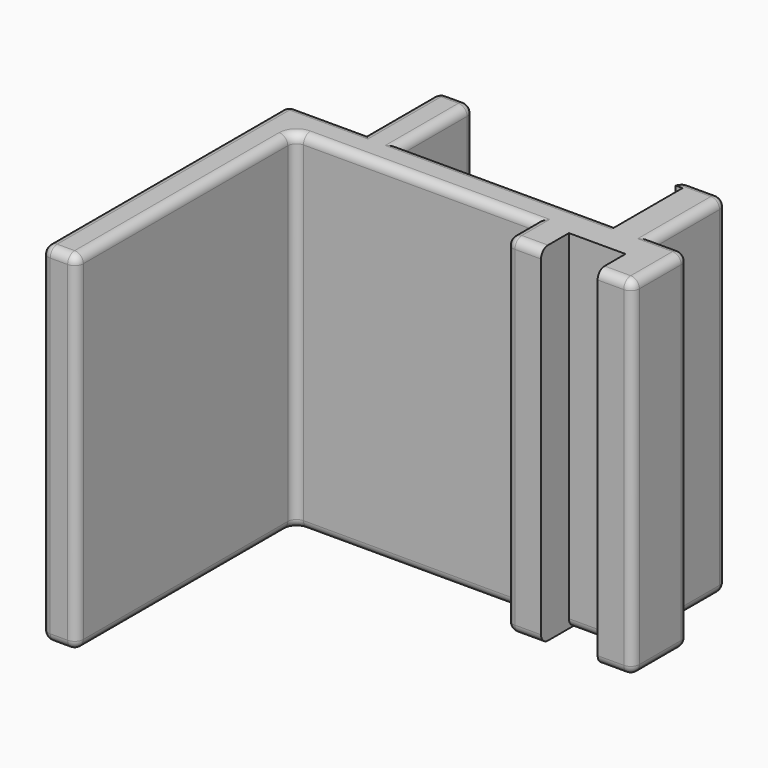
from build123d import *

# Parameters (mm, degrees)
F1_DEPTH = 40
F2_W     = 10.5
F2_H     = 17
F3_DEPTH = 4
F4_F1_R  = 1
F4_F2_R  = 1


with BuildPart() as f1:
    # F0 (on Top) → F1 (new body)
    with BuildSketch(Plane.XY):
        Polygon((-12.6578821212, 16.4037507206), (-21.6578821212, 16.4037507206), (-21.6578821212, -18.9613338028), (-17.6578821212, -18.9613338028), (-17.6578821212, 12.4037507206), (9.8421178788, 12.4037507206), (9.8421178788, 8.4037507206), (13.8421178788, 8.4037507206), (13.8421178788, 12.4037507206), (20.3421178788, 12.4037507206), (20.3421178788, 8.4037507206), (24.3421178788, 8.4037507206), (24.3421178788, 16.4037507206), (20.3421178788, 16.4037507206), (20.3421178788, 26.9037507206), (16.3421178788, 26.9037507206), (15.5421178788, 25.6037507206), (16.3421178788, 25.6037507206), (16.3421178788, 16.4037507206), (-8.6578821212, 16.4037507206), (-8.6578821212, 18.6537507206), (-12.6578821212, 18.6537507206), align=None)
    extrude(amount=F1_DEPTH)

    # F2 (on face) → F3 (join, through all)
    with BuildSketch(Plane(origin=(-12.6578821212, 0, 0), x_dir=(0, -1, 0), z_dir=(-1, 0, 0))):
        with Locations((-21.6537507206, 8.5)):
            Rectangle(F2_W, F2_H)
        with Locations((-21.6537507206, 31.5)):
            Rectangle(F2_W, F2_H)
    extrude(amount=-F3_DEPTH)

    # F4: fillet of radius 1 on 53 edges, made by hand

    # F4_f1
    f4_f1_edges = [f1.edges().sort_by_distance(p)[0] for p in [
        (-10.6578821212, 18.6537507206, 17),
        (-10.6578821212, 18.6537507206, 23),
        (-17.6578821212, 12.4037507206, 20),
    ]]
    fillet(f4_f1_edges, radius=F4_F1_R)

    # F4_f2
    f4_f2_edges = [f1.edges().sort_by_distance(p)[0] for p in [
        (20.3421178788, 26.9037507206, 20),
        (-10.6578821212, 26.9037507206, 17),
        (-10.6578821212, 26.9037507206, 23),
        (-10.6578821212, 26.9037507206, 0),
        (-10.6578821212, 26.9037507206, 40),
        (24.3421178788, 8.4037507206, 20),
        (9.8421178788, 8.4037507206, 20),
        (-21.6578821212, -18.9613338028, 20),
        (-12.6578821212, 21.6537507206, 40),
        (-12.6578821212, 21.6537507206, 0),
        (-12.6578821212, 26.9037507206, 8.5),
        (-12.6578821212, 26.9037507206, 31.5),
        (-17.1578821212, 16.4037507206, 0),
        (-17.1578821212, 16.4037507206, 40),
        (-21.6578821212, -1.2787915411, 40),
        (-21.6578821212, -1.2787915411, 0),
        (-19.6578821212, -18.9613338028, 40),
        (-19.6578821212, -18.9613338028, 0),
        (18.3421178788, 26.9037507206, 0),
        (18.3421178788, 26.9037507206, 40),
        (20.3421178788, 21.6537507206, 0),
        (20.3421178788, 21.6537507206, 40),
        (3.8421178788, 16.4037507206, 0),
        (3.8421178788, 16.4037507206, 40),
        (-3.4078821212, 12.4037507206, 0),
        (-3.4078821212, 12.4037507206, 40),
        (-17.6578821212, -18.9613338028, 20),
        (-8.6578821212, 21.6537507206, 0),
        (-8.6578821212, 26.9037507206, 8.5),
        (-8.6578821212, 26.9037507206, 31.5),
        (-8.6578821212, 21.6537507206, 40),
        (-12.6578821212, 23.2787507206, 17),
        (-8.6578821212, 23.2787507206, 17),
        (-8.6578821212, 18.6537507206, 20),
        (-12.6578821212, 18.6537507206, 20),
        (-12.6578821212, 23.2787507206, 23),
        (-8.6578821212, 23.2787507206, 23),
        (22.3421178788, 16.4037507206, 0),
        (24.3421178788, 12.4037507206, 0),
        (22.3421178788, 8.4037507206, 0),
        (9.8421178788, 10.4037507206, 0),
        (11.8421178788, 8.4037507206, 0),
        (17.0921178788, 12.4037507206, 0),
        (24.3421178788, 12.4037507206, 40),
        (22.3421178788, 8.4037507206, 40),
        (11.8421178788, 8.4037507206, 40),
        (9.8421178788, 10.4037507206, 40),
        (22.3421178788, 16.4037507206, 40),
        (24.3421178788, 16.4037507206, 20),
        (-21.6578821212, 16.4037507206, 20),
        (-8.6578821212, 18.9466439394, 22.7071067812),
        (-12.6578821212, 18.9466439394, 22.7071067812),
        (-12.6578821212, 18.9466439394, 17.2928932188),
        (-8.6578821212, 18.9466439394, 17.2928932188),
        (-17.3649889024, 12.1108575018, 40),
        (-17.3649889024, 12.1108575018, 0),
    ]]
    fillet(f4_f2_edges, radius=F4_F2_R)

    # F5 (on face) → F6 (revolve)
    with BuildSketch(Plane(origin=(0, 16.4037507206, 0), x_dir=(-1, 0, 0), z_dir=(0, 1, 0))):
        with BuildLine():
            Line((2.1578821212, 20), (-1.8421178788, 20))
            ThreePointArc((-1.8421178788, 20), (0.1578821212, 18), (2.1578821212, 20))
        make_face()
    revolve(axis=Axis((-0.1578821212, 16.4037507206, 20), (-1, 0, 0)))


solid = f1.part
